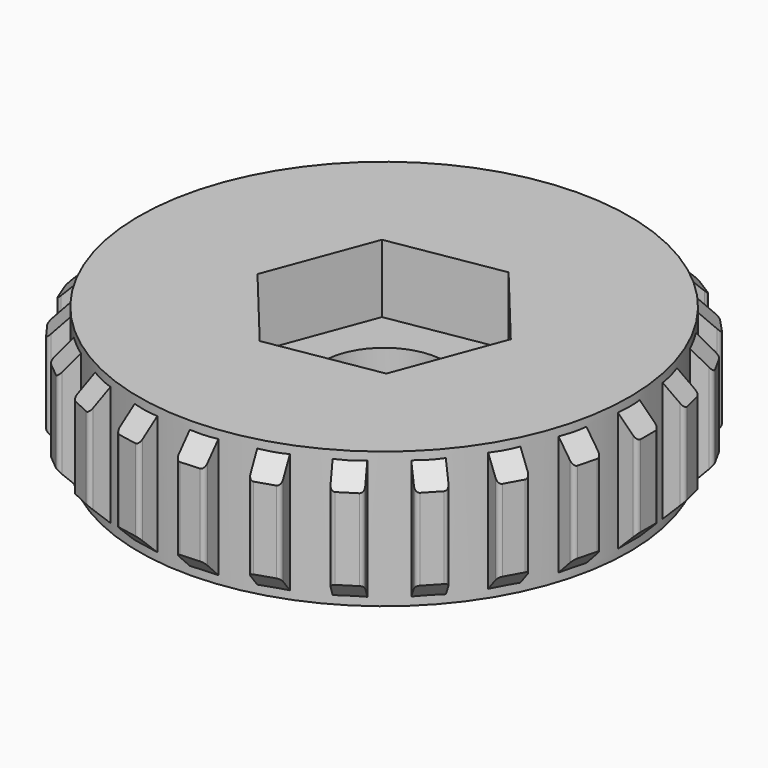
from build123d import *

# Parameters (mm, degrees)
F1_DEPTH    = 5
F2_R        = 0.15
F3_T1_DEPTH = 5.8433659759
F4_COUNT    = 25
F5_R        = 2.25
F6_DEPTH    = 5.001
F7_DEPTH    = 2.5


# Not quite as in the source:
# - a fillet or chamfer that OpenCascade refuses, or shapes differently, is made with other operations: its cross-section is extruded or revolved along the edge and cut away or added


with BuildPart() as f1:
    # F0 (on Top) → F1 (new body)
    with BuildSketch(Plane.XY):
        with BuildLine():
            ThreePointArc((8.9861003778, -0.5), (8.9965244234, -0.2500965811), (9, 0))
            ThreePointArc((9, 0), (8.9965244234, 0.2500965811), (8.9861003778, 0.5))
            ThreePointArc((8.9861003778, 0.5), (-9, 0), (8.9861003778, -0.5))
        make_face()
        with BuildLine():
            ThreePointArc((8.9861003778, 0.5), (8.9965244234, 0.2500965811), (9, 0))
            ThreePointArc((9, 0), (8.9965244234, -0.2500965811), (8.9861003778, -0.5))
            Line((8.9861003778, -0.5), (9.6871048306, -0.5))
            Line((9.6871048306, -0.5), (9.6871048306, 0.5))
            Line((9.6871048306, 0.5), (8.9861003778, 0.5))
        make_face()
    extrude(amount=F1_DEPTH)

    # F2
    f2_edges = [f1.edges().sort_by_distance(p)[0] for p in [
        (9.687105, -0.5, 2.5),
        (9.687105, 0.5, 2.5),
    ]]
    fillet(f2_edges, radius=F2_R)

    # F3: chamfer of 1 on 2 edges, made by hand

    # F3_s2 → F3_t1 (cut)
    with BuildSketch(Plane.XZ.offset(-2.921682988)):
        Polygon((8.6871048306, 0), (9.6871048306, 1), (9.6871048306, 0), align=None)
        Polygon((8.6871048306, 5), (9.6871048306, 4), (9.6871048306, 5), align=None)
    extrude(amount=F3_T1_DEPTH, mode=Mode.SUBTRACT)

    # F4: F1 ×25 about axis
    f4_axis = Axis((0, 0, 0), (0, 0, -1))


with BuildPart() as f1_1:
    add(f1.part)
    for i in range(1, F4_COUNT):
        add(f1.part.rotate(f4_axis, i * 360 / F4_COUNT))

    # F5 (on face) → F6 (cut, through all)
    with BuildSketch(Plane.XY.offset(5)):
        Circle(F5_R)
    extrude(amount=-F6_DEPTH, mode=Mode.SUBTRACT)

    # F5 (on face) → F7 (cut)
    with BuildSketch(Plane.XY.offset(5)):
        Polygon((2.6462685262, -3.205817039), (4.0994532587, 0.6888272494), (1.4531847326, 3.8946442884), (-2.6462685262, 3.205817039), (-4.0994532587, -0.6888272494), (-1.4531847326, -3.8946442884), align=None)
        Circle(F5_R, mode=Mode.SUBTRACT)
    extrude(amount=-F7_DEPTH, mode=Mode.SUBTRACT)


solid = f1_1.part
